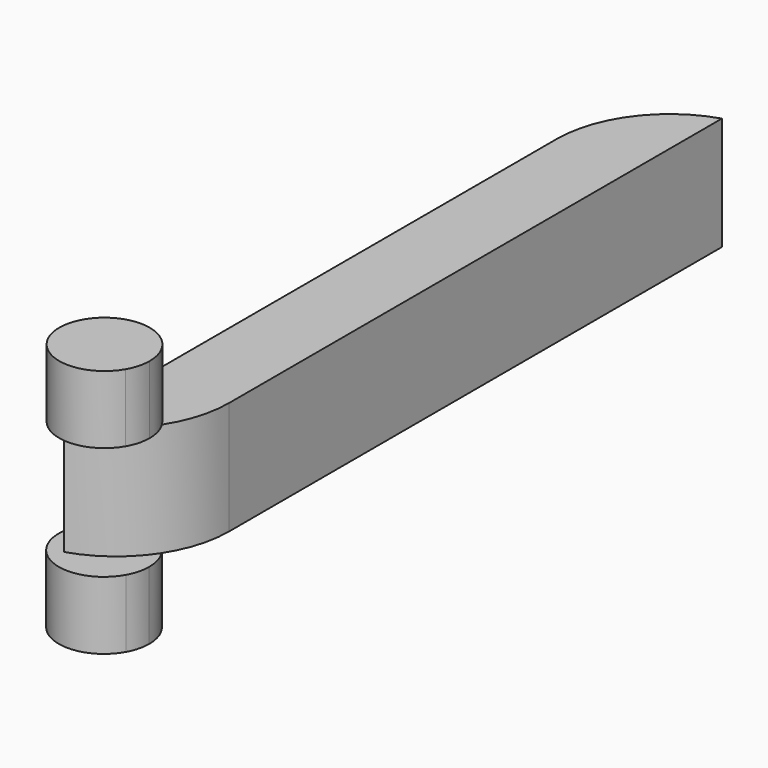
from build123d import *

# Parameters (mm, degrees)
F0_W        = 16
F0_H        = 2.5
F1_DEPTH    = 1.75
F4_DEPTH    = 1.5
F5_DEPTH    = 1.5
F6_T1_DEPTH = 14.4242400177
F6_T3_DEPTH = 2.5


# Not quite as in the source:
# - a fillet or chamfer that OpenCascade refuses, or shapes differently, is made with other operations: its cross-section is extruded or revolved along the edge and cut away or added


with BuildPart() as f1:
    # F0 (on Right) → F1 (new body)
    with BuildSketch(Plane.YZ):
        with Locations((8, 1.25)):
            Rectangle(F0_W, F0_H)
    extrude(amount=F1_DEPTH)

    # F3 (on face) → F4 (join)
    with BuildSketch(Plane.XY.offset(2.5)):
        with BuildLine():
            ThreePointArc((1.3660254038, 0), (1.4659258263, 0.2411809549), (1.5, 0.5))
            ThreePointArc((1.5, 0.5), (1, 1.3660254038), (0, 1.3660254038))
            Line((0, 1.3660254038), (0, 0))
            Line((0, 0), (1.3660254038, 0))
        make_face()
        with BuildLine():
            Line((0, 0), (0, 1.3660254038))
            ThreePointArc((0, 1.3660254038), (-0.2071067812, -0.2071067812), (1.3660254038, 0))
            Line((1.3660254038, 0), (0, 0))
        make_face()
    extrude(amount=F4_DEPTH)

    # F2 (on face) → F5 (join)
    with BuildSketch(Plane(origin=(0, 0, 0), x_dir=(1, 0, 0), z_dir=(0, 0, -1))):
        with BuildLine():
            ThreePointArc((0, -1.3527675268), (1, -1.3527675268), (1.5, -0.486742123))
            ThreePointArc((1.5, -0.486742123), (1.4678702674, -0.2352920375), (1.373545709, 0))
            Line((1.373545709, 0), (0, 0))
            Line((0, 0), (0, -1.3527675268))
        make_face()
        with BuildLine():
            Line((0, 0), (1.373545709, 0))
            ThreePointArc((1.373545709, 0), (-0.2016972955, 0.2257330733), (0, -1.3527675268))
            Line((0, -1.3527675268), (0, 0))
        make_face()
    extrude(amount=F5_DEPTH)

    # F6: fillet of radius 2.5 on 2 edges, made by hand

    # F6_s2 → F6_t1 (cut)
    with BuildSketch(Plane.XY.offset(-5.9621200089)):
        with BuildLine():
            ThreePointArc((0, 13.6151519965), (0.4844355629, 15.0941719422), (1.75, 16))
            Line((1.75, 16), (0, 16))
            Line((0, 16), (0, 13.6151519965))
        make_face()
    extrude(amount=F6_T1_DEPTH, mode=Mode.SUBTRACT)

    # F6_s4 → F6_t3 (cut)
    with BuildSketch(Plane.XY):
        with BuildLine():
            ThreePointArc((0, 0), (1.2655644371, 0.9058280578), (1.75, 2.3848480035))
            Line((1.75, 2.3848480035), (1.75, 0))
            Line((1.75, 0), (0, 0))
        make_face()
    extrude(amount=F6_T3_DEPTH, mode=Mode.SUBTRACT)


solid = f1.part
